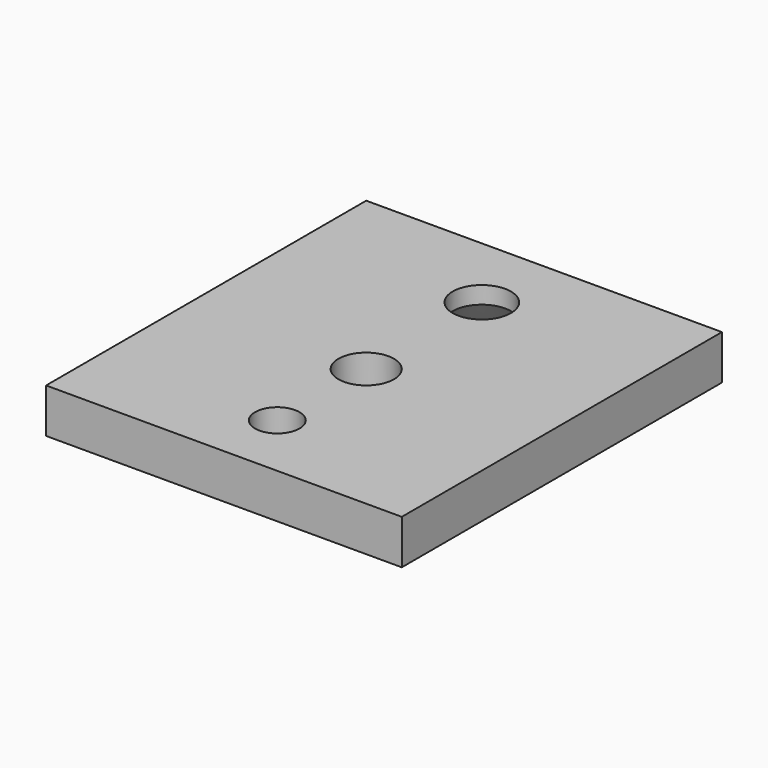
from build123d import *

# Parameters (mm, degrees)
F0_R           = 1.27
F1_DEPTH       = 12.7
F3_D           = 15.875
F5_D           = 16.66748
F5_CSINK_D     = 30.1752
F5_CSINK_ANGLE = 82
F7_D           = 12.7


# Not quite as in the source:
# - a feature names something its author has since deleted; it is built from what else it names


with BuildPart() as f1:
    # F0 (on Top) → F1 (new body)
    with BuildSketch(Plane.XY):
        Polygon((-2.5901260614, -38.4407882191), (-2.5901260614, 12.3592117809), (-2.5901260614, 63.1592117809), (-2.5901260614, 75.8592117809), (-104.1901260614, 75.8592117809), (-104.1901260614, 63.1592117809), (-104.1901260614, -38.4407882191), align=None)
        with Locations((-85.1401260614, 12.3592117809)):
            Circle(F0_R, mode=Mode.SUBTRACT)
        with Locations((-78.4163327398, -7.1792497576)):
            Circle(F0_R, mode=Mode.SUBTRACT)
        with Locations((-53.3901260614, -19.3907882191)):
            Circle(F0_R, mode=Mode.SUBTRACT)
        with Locations((-53.3901260614, 12.3592117809)):
            Circle(F0_R, mode=Mode.SUBTRACT)
        with Locations((-23.1804483045, 2.5899810116)):
            Circle(F0_R, mode=Mode.SUBTRACT)
        with BuildLine():
            ThreePointArc((-13.3851260614, 12.3592117809), (-12.1151260614, 13.6292117809), (-10.8451260614, 12.3592117809))
            ThreePointArc((-10.8451260614, 12.3592117809), (-12.1151260614, 11.0892117809), (-13.3851260614, 12.3592117809))
        make_face(mode=Mode.SUBTRACT)
        with Locations((-92.6627071454, 25.0592117809)):
            Circle(F0_R, mode=Mode.SUBTRACT)
        with Locations((-20.8560573795, 37.7592117809)):
            Circle(F0_R, mode=Mode.SUBTRACT)
        with Locations((-53.3901260614, 53.6342117809)):
            Circle(F0_R, mode=Mode.SUBTRACT)
        with Locations((-92.6627071454, 25.0592117809)):
            Circle(F0_R)
        with Locations((-85.1401260614, 12.3592117809)):
            Circle(F0_R)
        with Locations((-78.4163327398, -7.1792497576)):
            Circle(F0_R)
        with Locations((-23.1804483045, 2.5899810116)):
            Circle(F0_R)
        with Locations((-20.8560573795, 37.7592117809)):
            Circle(F0_R)
        with BuildLine():
            ThreePointArc((-13.3851260614, 12.3592117809), (-12.1151260614, 11.0892117809), (-10.8451260614, 12.3592117809))
            Line((-10.8451260614, 12.3592117809), (-13.3851260614, 12.3592117809))
        make_face()
        with BuildLine():
            Line((-13.3851260614, 12.3592117809), (-10.8451260614, 12.3592117809))
            ThreePointArc((-10.8451260614, 12.3592117809), (-12.1151260614, 13.6292117809), (-13.3851260614, 12.3592117809))
        make_face()
    extrude(amount=F1_DEPTH)

    # F3 (through all)
    with Locations(Plane.XY.offset(12.7)):
        with Locations((-53.3901260614, 12.3592117809)):
            Hole(F3_D / 2)

    # F5 (through all)
    with Locations(Plane(origin=(0, 0, 0), x_dir=(1, 0, 0), z_dir=(0, 0, -1))):
        with Locations((-53.3901260614, -53.6342117809)):
            CounterSinkHole(F5_D / 2, F5_CSINK_D / 2, counter_sink_angle=F5_CSINK_ANGLE)

    # F7 (through all)
    with Locations(Plane.XY.offset(12.7)):
        with Locations((-53.3901260614, -19.3907882191)):
            Hole(F7_D / 2)


solid = f1.part
